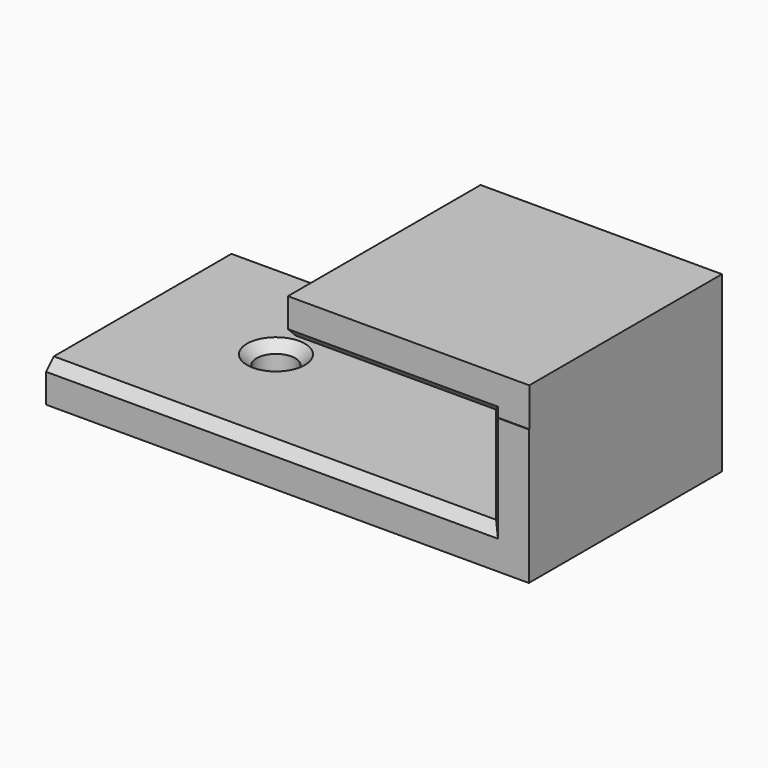
from build123d import *

# Parameters (mm, degrees)
F0_W           = 25
F0_H           = 12.5
F1_DEPTH       = 2
F2_W           = 2.0972218364
F2_H           = 12.5
F3_DEPTH       = 5
F4_W           = 12.5
F4_H           = 12.5694446266
F5_DEPTH       = 2
F6_SIZE        = 0.5
F8_D           = 2
F8_CSINK_D     = 3
F8_CSINK_ANGLE = 90
F9_DEPTH       = 0.1
F10_T4_DEPTH   = 13.4439057781
F10_T9_DEPTH   = 13.4439057781


# Not quite as in the source:
# - a fillet or chamfer that OpenCascade refuses, or shapes differently, is made with other operations: its cross-section is extruded or revolved along the edge and cut away or added


with BuildPart() as f1:
    # F0 (on Top) → F1 (new body)
    with BuildSketch(Plane.XY):
        Rectangle(F0_W, F0_H)
    extrude(amount=F1_DEPTH)

    # F2 (on face) → F3 (join)
    with BuildSketch(Plane.XY.offset(2)):
        with Locations((11.4513890818, 0)):
            Rectangle(F2_W, F2_H)
    extrude(amount=F3_DEPTH)

    # F4 (on face) → F5 (join)
    with BuildSketch(Plane.XY.offset(7)):
        with Locations((6.25, -0.0347223133)):
            Rectangle(F4_W, F4_H)
    extrude(amount=F5_DEPTH)

    # F6
    f6_edges = [f1.edges().sort_by_distance(p)[0] for p in [
        (10.402778, 6.25, 4.5),
        (-1.048611, 6.25, 2),
        (10.402778, -6.25, 4.5),
        (-1.048611, -6.25, 2),
        (5.201389, 6.25, 7),
    ]]
    chamfer(f6_edges, length=F6_SIZE)

    # F8 (through all)
    with Locations(Plane.XY.offset(2)):
        with Locations((-5.596134346, 0)):
            CounterSinkHole(F8_D / 2, F8_CSINK_D / 2, counter_sink_angle=F8_CSINK_ANGLE)

    # F9 (cut): a face of the model
    f9_faces = [f1.faces().sort_by_distance(p)[0] for p in [
        (6.25, -6.3194446266, 8),
    ]]
    extrude(f9_faces, amount=-F9_DEPTH, mode=Mode.SUBTRACT)

    # F10: chamfer of 0.5 on 1 edges, made by hand


with BuildPart() as f10_tool2:
    # F10_s3 → F10_t4 (new body)
    with BuildSketch(Plane.YZ.offset(-1.285841494)):
        Polygon((-5.7194446266, 7), (-6.2194446266, 7.5), (-6.2194446266, 7), align=None)
    extrude(amount=F10_T4_DEPTH)

    split(bisect_by=Plane(origin=(2.3263890818, 2.3263890818, 0), x_dir=(0, 0, 1), z_dir=(-0.7071067812, -0.7071067812, 0)), keep=Keep.TOP)


with BuildPart() as f1_1:
    add(f1.part)

    # F10_t1: cut F10_tool2
    add(f10_tool2.part, mode=Mode.SUBTRACT)


with BuildPart() as f10_tool7:
    # F10_s8 → F10_t9 (new body)
    with BuildSketch(Plane.YZ.offset(-1.285841494)):
        Polygon((-5.7194446266, 7), (-6.2194446266, 7.5), (-6.2194446266, 7), align=None)
    extrude(amount=F10_T9_DEPTH)

    split(bisect_by=Plane.YZ.offset(10.4027781636), keep=Keep.BOTTOM)


with BuildPart() as f1_2:
    add(f1_1.part)

    # F10_t6: cut F10_tool7
    add(f10_tool7.part, mode=Mode.SUBTRACT)


solid = f1_2.part
